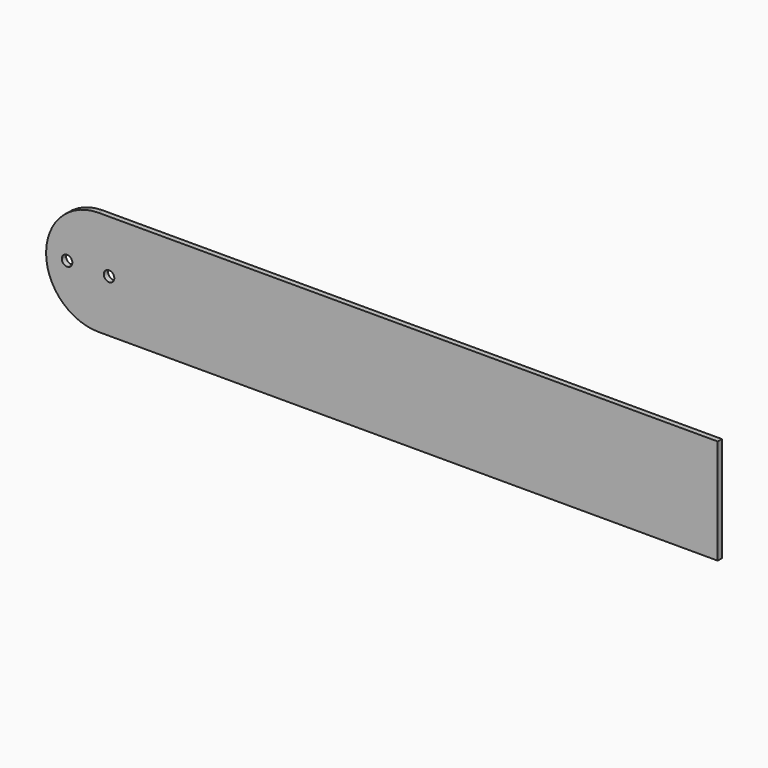
from build123d import *

# Parameters (mm, degrees)
F1_DEPTH = 3.175


# Not quite as in the source:
# - a feature names something its author has since deleted; it is built from what else it names


with BuildPart() as f1:
    # F0 (on Front) → F1 (new body)
    with BuildSketch(Plane.XZ):
        with BuildLine():
            ThreePointArc((0, 31.75), (9.2993596973, 9.2993596973), (31.75, 0))
            Line((31.75, 0), (329.6745226565, 0))
            ThreePointArc((329.6745226565, 0), (322.395318302, 11.9320738166), (318.7033258065, 25.4128153768))
            ThreePointArc((318.7033258065, 25.4128153768), (311.9501, 31.75), (318.7033258065, 38.0871846232))
            ThreePointArc((318.7033258065, 38.0871846232), (322.395318302, 51.5679261834), (329.6745226565, 63.5))
            Line((329.6745226565, 63.5), (31.75, 63.5))
            ThreePointArc((31.75, 63.5), (9.2993596973, 54.2006403027), (0, 31.75))
        make_face()
        with BuildLine():
            ThreePointArc((12.8984375, 28.5812072396), (10.5262260999, 29.4358409667), (9.525, 31.75))
            ThreePointArc((9.525, 31.75), (10.5262260999, 34.0641590333), (12.8984375, 34.9187927604))
            ThreePointArc((12.8984375, 34.9187927604), (39.6875, 57.1003420835), (63.5, 31.75))
            ThreePointArc((63.5, 31.75), (39.6875, 6.3996579165), (12.8984375, 28.5812072396))
        make_face(mode=Mode.SUBTRACT)
        with BuildLine():
            ThreePointArc((318.7033258065, 25.4128153768), (322.395318302, 11.9320738166), (329.6745226565, 0))
            Line((329.6745226565, 0), (406.4, 0))
            Line((406.4, 0), (406.4, 63.5))
            Line((406.4, 63.5), (329.6745226565, 63.5))
            ThreePointArc((329.6745226565, 63.5), (322.395318302, 51.5679261834), (318.7033258065, 38.0871846232))
            ThreePointArc((318.7033258065, 38.0871846232), (322.9305958628, 36.0952281948), (324.6501, 31.75))
            ThreePointArc((324.6501, 31.75), (322.9305958628, 27.4047718052), (318.7033258065, 25.4128153768))
        make_face()
        with BuildLine():
            ThreePointArc((63.5, 31.75), (39.6875, 57.1003420835), (12.8984375, 34.9187927604))
            ThreePointArc((12.8984375, 34.9187927604), (15.0141590333, 33.9237739001), (15.875, 31.75))
            ThreePointArc((15.875, 31.75), (15.0141590333, 29.5762260999), (12.8984375, 28.5812072396))
            ThreePointArc((12.8984375, 28.5812072396), (39.6875, 6.3996579165), (63.5, 31.75))
        make_face()
        with BuildLine():
            ThreePointArc((41.275, 31.75), (38.1, 28.575), (34.925, 31.75))
            ThreePointArc((34.925, 31.75), (38.1, 34.925), (41.275, 31.75))
        make_face(mode=Mode.SUBTRACT)
        with BuildLine():
            ThreePointArc((318.7033258065, 38.0871846232), (311.9501, 31.75), (318.7033258065, 25.4128153768))
            ThreePointArc((318.7033258065, 25.4128153768), (318.3001, 31.75), (318.7033258065, 38.0871846232))
        make_face()
        with BuildLine():
            ThreePointArc((318.7033258065, 38.0871846232), (318.3001, 31.75), (318.7033258065, 25.4128153768))
            ThreePointArc((318.7033258065, 25.4128153768), (322.9305958628, 27.4047718052), (324.6501, 31.75))
            ThreePointArc((324.6501, 31.75), (322.9305958628, 36.0952281948), (318.7033258065, 38.0871846232))
        make_face()
    extrude(amount=F1_DEPTH)


solid = f1.part
